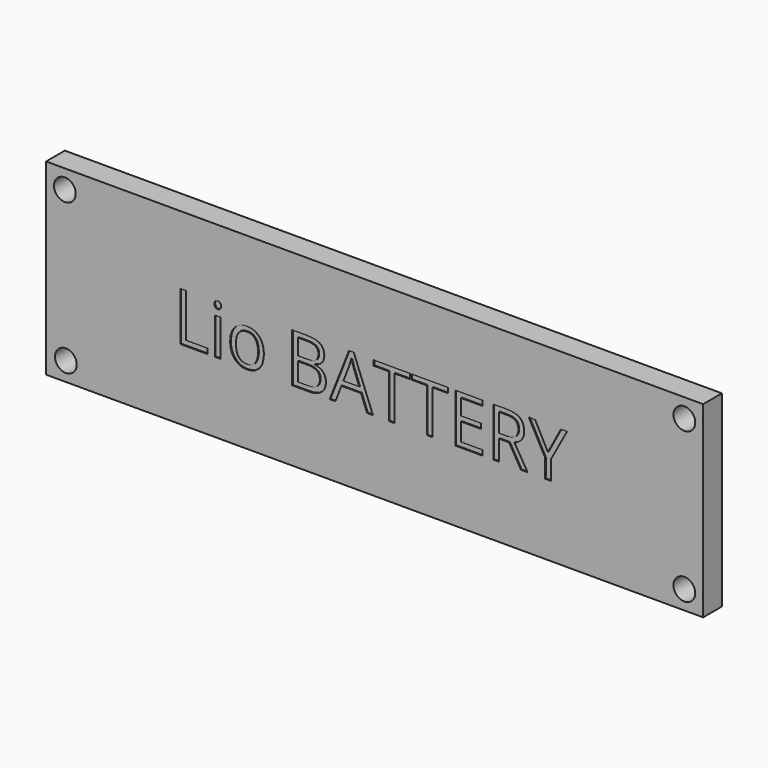
from build123d import *

# Parameters (mm, degrees)
F0_W         = 88.9
F0_H         = 25.4
F0_R         = 1.4732
F0_W_2       = 0.7499087036
F0_H_2       = 4.9488194792
F1_DEPTH     = 3.175
F0_TEXT_SIZE = 9.2474290998
F2_DEPTH     = 3.048


# Not quite as in the source:
# - Text() gives the source's letters only with a copy of the font that has no kerning and outlines rounded to 1/6400 em; it was checked with that copy


with BuildPart() as f1:
    # F0 (on Front) → F1 (new body)
    with BuildSketch(Plane.XZ):
        with Locations((7.4413009771, 13.4895089843)):
            Rectangle(F0_W, F0_H)
        with Locations((-34.3324406526, 3.3295089843)):
            Circle(F0_R, mode=Mode.SUBTRACT)
        with Locations((49.3513009771, 3.3295089843)):
            Circle(F0_R, mode=Mode.SUBTRACT)
        with BuildLine():
            Line((46.8211543225, 2.3461586478), (-31.9188456775, 2.3461586478))
            Line((-31.9188456775, 2.3461586478), (-31.9188456775, 3.2986586478))
            ThreePointArc((-31.9188456775, 3.2986586478), (-32.6627944533, 5.094709872), (-34.4588456775, 5.8386586478))
            Line((-34.4588456775, 5.8386586478), (-35.4113456775, 5.8386586478))
            Line((-35.4113456775, 5.8386586478), (-35.4113456775, 21.0786586478))
            Line((-35.4113456775, 21.0786586478), (-34.4588456775, 21.0786586478))
            ThreePointArc((-34.4588456775, 21.0786586478), (-32.6627944533, 21.8226074236), (-31.9188456775, 23.6186586478))
            Line((-31.9188456775, 23.6186586478), (-31.9188456775, 24.5711586478))
            Line((-31.9188456775, 24.5711586478), (46.8211543225, 24.5711586478))
            Line((46.8211543225, 24.5711586478), (46.8211543225, 23.6186586478))
            ThreePointArc((46.8211543225, 23.6186586478), (47.5651030982, 21.8226074236), (49.3611543225, 21.0786586478))
            Line((49.3611543225, 21.0786586478), (50.3136543225, 21.0786586478))
            Line((50.3136543225, 21.0786586478), (50.3136543225, 5.8386586478))
            Line((50.3136543225, 5.8386586478), (49.3581127419, 5.8386586478))
            ThreePointArc((49.3581127419, 5.8386586478), (47.6065470167, 5.1381198489), (46.8211543225, 3.4229244041))
            Line((46.8211543225, 3.4229244041), (46.8211543225, 2.3461586478))
        make_face(mode=Mode.SUBTRACT)
        with Locations((-34.4686990229, 23.6495089843)):
            Circle(F0_R, mode=Mode.SUBTRACT)
        with Locations((49.3513009771, 23.6495089843)):
            Circle(F0_R, mode=Mode.SUBTRACT)
        with BuildLine():
            Line((-31.9188456775, 3.2986586478), (-31.9188456775, 2.3461586478))
            Line((-31.9188456775, 2.3461586478), (46.8211543225, 2.3461586478))
            Line((46.8211543225, 2.3461586478), (46.8211543225, 3.4229244041))
            ThreePointArc((46.8211543225, 3.4229244041), (47.6065470167, 5.1381198489), (49.3581127419, 5.8386586478))
            Line((49.3581127419, 5.8386586478), (50.3136543225, 5.8386586478))
            Line((50.3136543225, 5.8386586478), (50.3136543225, 21.0786586478))
            Line((50.3136543225, 21.0786586478), (49.3611543225, 21.0786586478))
            ThreePointArc((49.3611543225, 21.0786586478), (47.5651030982, 21.8226074236), (46.8211543225, 23.6186586478))
            Line((46.8211543225, 23.6186586478), (46.8211543225, 24.5711586478))
            Line((46.8211543225, 24.5711586478), (-31.9188456775, 24.5711586478))
            Line((-31.9188456775, 24.5711586478), (-31.9188456775, 23.6186586478))
            ThreePointArc((-31.9188456775, 23.6186586478), (-32.6627944533, 21.8226074236), (-34.4588456775, 21.0786586478))
            Line((-34.4588456775, 21.0786586478), (-35.4113456775, 21.0786586478))
            Line((-35.4113456775, 21.0786586478), (-35.4113456775, 5.8386586478))
            Line((-35.4113456775, 5.8386586478), (-34.4588456775, 5.8386586478))
            ThreePointArc((-34.4588456775, 5.8386586478), (-32.6627944533, 5.094709872), (-31.9188456775, 3.2986586478))
        make_face()
        with Locations((-13.7870462985, 12.8233742221)):
            Rectangle(F0_W_2, F0_H_2, mode=Mode.SUBTRACT)
        with BuildLine():
            add(Edge.make_bspline(
                [(-8.1634534772, 14.6974235256), (-7.5515337547, 14.0060337093), (-7.5515337547, 12.8284314099)],
                knots=[0, 0, 0, 1, 1, 1], degree=2))
            add(Edge.make_bspline(
                [(-7.5515337547, 12.8284314099), (-7.5515337547, 11.6175961622), (-8.1605636556, 10.9377656323)],
                knots=[0, 0, 0, 1, 1, 1], degree=2))
            add(Edge.make_bspline(
                [(-8.1605636556, 10.9377656323), (-8.7695935565, 10.2579351023), (-9.8446071893, 10.2579351023)],
                knots=[0, 0, 0, 1, 1, 1], degree=2))
            add(Edge.make_bspline(
                [(-9.8446071893, 10.2579351023), (-10.5092661559, 10.2579351023), (-11.0236543995, 10.5700358345)],
                knots=[0, 0, 0, 1, 1, 1], degree=2))
            add(Edge.make_bspline(
                [(-11.0236543995, 10.5700358345), (-11.5380426432, 10.8821365666), (-11.8183553378, 11.4644356177)],
                knots=[0, 0, 0, 1, 1, 1], degree=2))
            add(Edge.make_bspline(
                [(-11.8183553378, 11.4644356177), (-12.0986680324, 12.0467346688), (-12.0986680324, 12.8284314099)],
                knots=[0, 0, 0, 1, 1, 1], degree=2))
            add(Edge.make_bspline(
                [(-12.0986680324, 12.8284314099), (-12.0986680324, 14.0378217469), (-11.4932504085, 14.7133175444)],
                knots=[0, 0, 0, 1, 1, 1], degree=2))
            add(Edge.make_bspline(
                [(-11.4932504085, 14.7133175444), (-10.8878327846, 15.3888133419), (-9.8128191518, 15.3888133419)],
                knots=[0, 0, 0, 1, 1, 1], degree=2))
            add(Edge.make_bspline(
                [(-9.8128191518, 15.3888133419), (-8.7753731997, 15.3888133419), (-8.1634534772, 14.6974235256)],
                knots=[0, 0, 0, 1, 1, 1], degree=2))
        make_face(mode=Mode.SUBTRACT)
        Polygon((-15.1691034757, 10.3489644825), (-18.8492912752, 10.3489644825), (-18.8492912752, 16.9507619133), (-18.0820436421, 16.9507619133), (-18.0820436421, 11.0439665758), (-15.1691034757, 11.0439665758), align=None, mode=Mode.SUBTRACT)
        with BuildLine():
            add(Edge.make_bspline(
                [(-14.0991470306, 16.2615394632), (-14.2255767253, 16.3858017917), (-14.2255767253, 16.6386611812)],
                knots=[0, 0, 0, 1, 1, 1], degree=2))
            add(Edge.make_bspline(
                [(-14.2255767253, 16.6386611812), (-14.2255767253, 16.895855303), (-14.0991470306, 17.0157828992)],
                knots=[0, 0, 0, 1, 1, 1], degree=2))
            add(Edge.make_bspline(
                [(-14.0991470306, 17.0157828992), (-13.9727173359, 17.1357104953), (-13.7819891107, 17.1357104953)],
                knots=[0, 0, 0, 1, 1, 1], degree=2))
            add(Edge.make_bspline(
                [(-13.7819891107, 17.1357104953), (-13.6013752611, 17.1357104953), (-13.470610834, 17.013615533)],
                knots=[0, 0, 0, 1, 1, 1], degree=2))
            add(Edge.make_bspline(
                [(-13.470610834, 17.013615533), (-13.3398464069, 16.8915205706), (-13.3398464069, 16.6386611812)],
                knots=[0, 0, 0, 1, 1, 1], degree=2))
            add(Edge.make_bspline(
                [(-13.3398464069, 16.6386611812), (-13.3398464069, 16.3858017917), (-13.470610834, 16.2615394632)],
                knots=[0, 0, 0, 1, 1, 1], degree=2))
            add(Edge.make_bspline(
                [(-13.470610834, 16.2615394632), (-13.6013752611, 16.1372771347), (-13.7819891107, 16.1372771347)],
                knots=[0, 0, 0, 1, 1, 1], degree=2))
            add(Edge.make_bspline(
                [(-13.7819891107, 16.1372771347), (-13.9727173359, 16.1372771347), (-14.0991470306, 16.2615394632)],
                knots=[0, 0, 0, 1, 1, 1], degree=2))
        make_face(mode=Mode.SUBTRACT)
        with BuildLine():
            Line((-3.7210752323, 10.3489644825), (-3.7210752323, 16.9507619133))
            Line((-3.7210752323, 16.9507619133), (-1.8556953936, 16.9507619133))
            add(Edge.make_bspline(
                [(-1.8556953936, 16.9507619133), (-0.5422714793, 16.9507619133), (0.0450847596, 16.5577461766)],
                knots=[0, 0, 0, 1, 1, 1], degree=2))
            add(Edge.make_bspline(
                [(0.0450847596, 16.5577461766), (0.6324409985, 16.1647304398), (0.6324409985, 15.3165678021)],
                knots=[0, 0, 0, 1, 1, 1], degree=2))
            add(Edge.make_bspline(
                [(0.6324409985, 15.3165678021), (0.6324409985, 14.7284891078), (0.3051687031, 14.3470326574)],
                knots=[0, 0, 0, 1, 1, 1], degree=2))
            add(Edge.make_bspline(
                [(0.3051687031, 14.3470326574), (-0.0221035924, 13.965576207), (-0.6506397891, 13.8528731649)],
                knots=[0, 0, 0, 1, 1, 1], degree=2))
            Line((-0.6506397891, 13.8528731649), (-0.6506397891, 13.8080809302))
            add(Edge.make_bspline(
                [(-0.6506397891, 13.8080809302), (0.8535123505, 13.5508868083), (0.8535123505, 12.2273485184)],
                knots=[0, 0, 0, 1, 1, 1], degree=2))
            add(Edge.make_bspline(
                [(0.8535123505, 12.2273485184), (0.8535123505, 11.3430631108), (0.2553192806, 10.8460137967)],
                knots=[0, 0, 0, 1, 1, 1], degree=2))
            add(Edge.make_bspline(
                [(0.2553192806, 10.8460137967), (-0.3428737893, 10.3489644825), (-1.4178874222, 10.3489644825)],
                knots=[0, 0, 0, 1, 1, 1], degree=2))
            Line((-1.4178874222, 10.3489644825), (-3.7210752323, 10.3489644825))
        make_face(mode=Mode.SUBTRACT)
        Polygon((7.2154545889, 10.3489644825), (6.4207536507, 10.3489644825), (5.5985994073, 12.4484198704), (2.9529677383, 12.4484198704), (2.1409278704, 10.3489644825), (1.3635658617, 10.3489644825), (3.9730747608, 16.9782152184), (4.618949887, 16.9782152184), align=None, mode=Mode.SUBTRACT)
        Polygon((10.1544031497, 16.2687640172), (10.1544031497, 10.3489644825), (9.3871555166, 10.3489644825), (9.3871555166, 16.2687640172), (7.2963695936, 16.2687640172), (7.2963695936, 16.9507619133), (12.2451890727, 16.9507619133), (12.2451890727, 16.2687640172), align=None, mode=Mode.SUBTRACT)
        Polygon((15.2708322813, 16.2687640172), (15.2708322813, 10.3489644825), (14.5035846482, 10.3489644825), (14.5035846482, 16.2687640172), (12.4127987252, 16.2687640172), (12.4127987252, 16.9507619133), (17.3616182043, 16.9507619133), (17.3616182043, 16.2687640172), align=None, mode=Mode.SUBTRACT)
        Polygon((22.0359046321, 11.035297111), (22.0359046321, 10.3489644825), (18.3557168326, 10.3489644825), (18.3557168326, 16.9507619133), (22.0359046321, 16.9507619133), (22.0359046321, 16.2687640172), (19.1229644657, 16.2687640172), (19.1229644657, 14.1418553242), (21.8596255149, 14.1418553242), (21.8596255149, 13.4641921605), (19.1229644657, 13.4641921605), (19.1229644657, 11.035297111), align=None, mode=Mode.SUBTRACT)
        with BuildLine():
            Line((25.6438468918, 13.0942949965), (24.2654019916, 13.0942949965))
            Line((24.2654019916, 13.0942949965), (24.2654019916, 10.3489644825))
            Line((24.2654019916, 10.3489644825), (23.4981543585, 10.3489644825))
            Line((23.4981543585, 10.3489644825), (23.4981543585, 16.9507619133))
            Line((23.4981543585, 16.9507619133), (25.3086275869, 16.9507619133))
            add(Edge.make_bspline(
                [(25.3086275869, 16.9507619133), (26.5237975671, 16.9507619133), (27.103929252, 16.4855006367)],
                knots=[0, 0, 0, 1, 1, 1], degree=2))
            add(Edge.make_bspline(
                [(27.103929252, 16.4855006367), (27.6840609369, 16.0202393601), (27.6840609369, 15.0853820746)],
                knots=[0, 0, 0, 1, 1, 1], degree=2))
            add(Edge.make_bspline(
                [(27.6840609369, 15.0853820746), (27.6840609369, 13.7762928926), (26.3561879146, 13.3153663485)],
                knots=[0, 0, 0, 1, 1, 1], degree=2))
            Line((26.3561879146, 13.3153663485), (28.1493222135, 10.3489644825))
            Line((28.1493222135, 10.3489644825), (27.2419182331, 10.3489644825))
            Line((27.2419182331, 10.3489644825), (25.6438468918, 13.0942949965))
        make_face(mode=Mode.SUBTRACT)
        Polygon((29.1463106633, 16.9507619133), (30.8946527275, 13.6491407425), (32.6545540781, 16.9507619133), (33.4853777862, 16.9507619133), (31.2818888211, 12.9093464145), (31.2818888211, 10.3489644825), (30.5059717232, 10.3489644825), (30.5059717232, 12.8732236446), (28.3068174904, 16.9507619133), align=None, mode=Mode.SUBTRACT)
    extrude(amount=F1_DEPTH)


with BuildPart() as f1b:
    # F0 (on Front) → F1, piece 2 (new body)
    with BuildSketch(Plane.XZ):
        with BuildLine():
            add(Edge.make_bspline(
                [(-10.9463516719, 14.268285019), (-11.3213060237, 13.7849623574), (-11.3213060237, 12.8284314099)],
                knots=[0, 0, 0, 1, 1, 1], degree=2))
            add(Edge.make_bspline(
                [(-11.3213060237, 12.8284314099), (-11.3213060237, 11.8791250164), (-10.9420169395, 11.3827981577)],
                knots=[0, 0, 0, 1, 1, 1], degree=2))
            add(Edge.make_bspline(
                [(-10.9420169395, 11.3827981577), (-10.5627278554, 10.886471299), (-9.8272682598, 10.886471299)],
                knots=[0, 0, 0, 1, 1, 1], degree=2))
            add(Edge.make_bspline(
                [(-9.8272682598, 10.886471299), (-9.0903637534, 10.886471299), (-8.708907303, 11.3806307915)],
                knots=[0, 0, 0, 1, 1, 1], degree=2))
            add(Edge.make_bspline(
                [(-8.708907303, 11.3806307915), (-8.3274508527, 11.874790284), (-8.3274508527, 12.8284314099)],
                knots=[0, 0, 0, 1, 1, 1], degree=2))
            add(Edge.make_bspline(
                [(-8.3274508527, 12.8284314099), (-8.3274508527, 13.7719581603), (-8.708907303, 14.2617829204)],
                knots=[0, 0, 0, 1, 1, 1], degree=2))
            add(Edge.make_bspline(
                [(-8.708907303, 14.2617829204), (-9.0903637534, 14.7516076805), (-9.8359377245, 14.7516076805)],
                knots=[0, 0, 0, 1, 1, 1], degree=2))
            add(Edge.make_bspline(
                [(-9.8359377245, 14.7516076805), (-10.5713973201, 14.7516076805), (-10.9463516719, 14.268285019)],
                knots=[0, 0, 0, 1, 1, 1], degree=2))
        make_face()
    extrude(amount=F1_DEPTH)


with BuildPart() as f1c:
    # F0 (on Front) → F1, piece 3 (new body)
    with BuildSketch(Plane.XZ):
        with BuildLine():
            Line((-2.9538275992, 16.2861029468), (-2.9538275992, 14.1245163947))
            Line((-2.9538275992, 14.1245163947), (-1.689530652, 14.1245163947))
            add(Edge.make_bspline(
                [(-1.689530652, 14.1245163947), (-0.8760458734, 14.1245163947), (-0.5191529065, 14.3795431503)],
                knots=[0, 0, 0, 1, 1, 1], degree=2))
            add(Edge.make_bspline(
                [(-0.5191529065, 14.3795431503), (-0.1622599397, 14.634569906), (-0.1622599397, 15.238542619)],
                knots=[0, 0, 0, 1, 1, 1], degree=2))
            add(Edge.make_bspline(
                [(-0.1622599397, 15.238542619), (-0.1622599397, 15.7948332758), (-0.5596104089, 16.0404681113)],
                knots=[0, 0, 0, 1, 1, 1], degree=2))
            add(Edge.make_bspline(
                [(-0.5596104089, 16.0404681113), (-0.956960878, 16.2861029468), (-1.8239073561, 16.2861029468)],
                knots=[0, 0, 0, 1, 1, 1], degree=2))
            Line((-1.8239073561, 16.2861029468), (-2.9538275992, 16.2861029468))
        make_face()
    extrude(amount=F1_DEPTH)


with BuildPart() as f1d:
    # F0 (on Front) → F1, piece 4 (new body)
    with BuildSketch(Plane.XZ):
        with BuildLine():
            Line((-1.6389587741, 13.4743065361), (-2.9538275992, 13.4743065361))
            Line((-2.9538275992, 13.4743065361), (-2.9538275992, 11.0035090735))
            Line((-2.9538275992, 11.0035090735), (-1.575382699, 11.0035090735))
            add(Edge.make_bspline(
                [(-1.575382699, 11.0035090735), (-0.7763470284, 11.0035090735), (-0.3724944607, 11.312719984)],
                knots=[0, 0, 0, 1, 1, 1], degree=2))
            add(Edge.make_bspline(
                [(-0.3724944607, 11.312719984), (0.0313581071, 11.6219308946), (0.0313581071, 12.2822551287)],
                knots=[0, 0, 0, 1, 1, 1], degree=2))
            add(Edge.make_bspline(
                [(0.0313581071, 12.2822551287), (0.0313581071, 12.8963422174), (-0.3818863808, 13.1853243767)],
                knots=[0, 0, 0, 1, 1, 1], degree=2))
            add(Edge.make_bspline(
                [(-0.3818863808, 13.1853243767), (-0.7951308687, 13.4743065361), (-1.6389587741, 13.4743065361)],
                knots=[0, 0, 0, 1, 1, 1], degree=2))
        make_face()
    extrude(amount=F1_DEPTH)


with BuildPart() as f1e:
    # F0 (on Front) → F1, piece 5 (new body)
    with BuildSketch(Plane.XZ):
        with BuildLine():
            Line((3.2246109681, 13.1390872312), (5.3601891258, 13.1390872312))
            Line((5.3601891258, 13.1390872312), (4.5914965819, 15.1850809196))
            add(Edge.make_bspline(
                [(4.5914965819, 15.1850809196), (4.4426707698, 15.5737619239), (4.2851754929, 16.1372771347)],
                knots=[0, 0, 0, 1, 1, 1], degree=2))
            add(Edge.make_bspline(
                [(4.2851754929, 16.1372771347), (4.185476648, 15.7038038956), (4.000528066, 15.1850809196)],
                knots=[0, 0, 0, 1, 1, 1], degree=2))
            Line((4.000528066, 15.1850809196), (3.2246109681, 13.1390872312))
        make_face()
    extrude(amount=F1_DEPTH)


with BuildPart() as f1f:
    # F0 (on Front) → F1, piece 6 (new body)
    with BuildSketch(Plane.XZ):
        with BuildLine():
            Line((24.2654019916, 16.277433482), (24.2654019916, 13.7531743199))
            Line((24.2654019916, 13.7531743199), (25.3187419625, 13.7531743199))
            add(Edge.make_bspline(
                [(25.3187419625, 13.7531743199), (26.1307818303, 13.7531743199), (26.5100709145, 14.076111883)],
                knots=[0, 0, 0, 1, 1, 1], degree=2))
            add(Edge.make_bspline(
                [(26.5100709145, 14.076111883), (26.8893599987, 14.3990494461), (26.8893599987, 15.0449245723)],
                knots=[0, 0, 0, 1, 1, 1], degree=2))
            add(Edge.make_bspline(
                [(26.8893599987, 15.0449245723), (26.8893599987, 15.6994691632), (26.5035688159, 15.9884513226)],
                knots=[0, 0, 0, 1, 1, 1], degree=2))
            add(Edge.make_bspline(
                [(26.5035688159, 15.9884513226), (26.1177776332, 16.277433482), (25.2638353522, 16.277433482)],
                knots=[0, 0, 0, 1, 1, 1], degree=2))
            Line((25.2638353522, 16.277433482), (24.2654019916, 16.277433482))
        make_face()
    extrude(amount=F1_DEPTH)


with BuildPart() as f2:
    # F0 (on Front) → F2 (new body)
    with BuildSketch(Plane.XZ):
        with Locations((-19.7566952556, 10.3489644825)):
            Text('Lio BATTERY', F0_TEXT_SIZE, font='Open Sans', text_align=(TextAlign.LEFT, TextAlign.BOTTOM))
    extrude(amount=F2_DEPTH)


solid = Compound([f1.part, f1b.part, f1c.part, f1d.part, f1e.part, f1f.part, f2.part])
